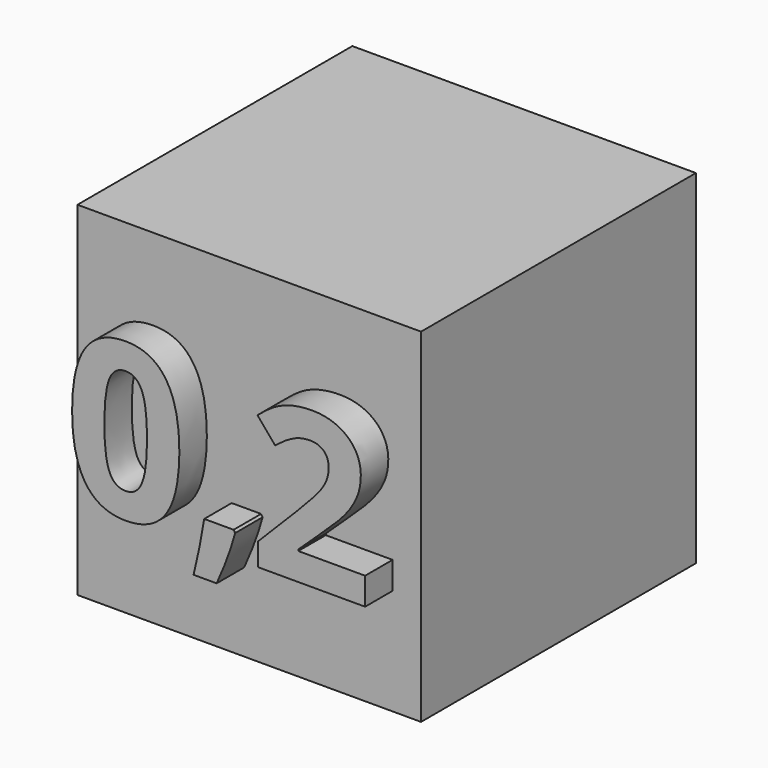
from build123d import *

# Parameters (mm, degrees)
F0_W         = 20
F0_H         = 20
F1_DEPTH     = 20
F2_TEXT_SIZE = 12.506831101
F3_DEPTH     = 2


# Not quite as in the source:
# - Text() gives the source's letters only with a copy of the font that has no kerning and outlines rounded to 1/6400 em; it was checked with that copy


with BuildPart() as f1:
    # F0 (on Front) → F1 (new body)
    with BuildSketch(Plane.XZ):
        with Locations((-10, 10)):
            Rectangle(F0_W, F0_H)
    extrude(amount=F1_DEPTH)

    # F2 (on face) → F3 (join)
    with BuildSketch(Plane.XZ.offset(20)):
        with Locations((-19.1631969064, 6.1782258563)):
            Text('0,2', F2_TEXT_SIZE, font='Open Sans', font_style=FontStyle.BOLD, text_align=(TextAlign.LEFT, TextAlign.BOTTOM))
    extrude(amount=F3_DEPTH)


solid = f1.part
